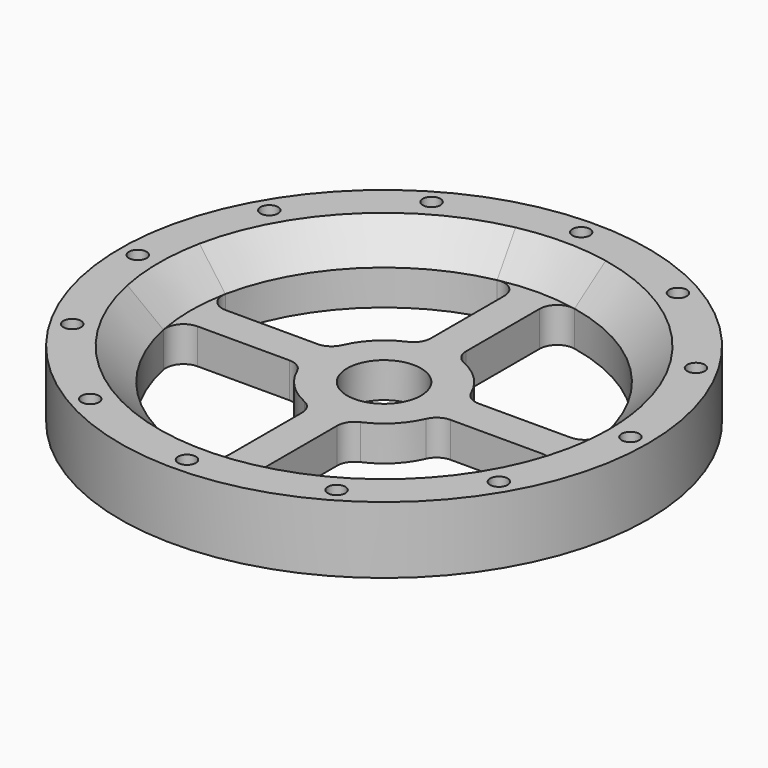
from build123d import *

# Parameters (mm, degrees)
F0_R     = 75
F0_R_2   = 2.5
F0_R_3   = 10.5
F1_DEPTH = 10
F2_R     = 5
F3_R     = 75
F3_R_2   = 2.5
F4_DEPTH = 9
F5_SIZE  = 8.99999


# Not quite as in the source:
# - a fillet or chamfer is up to 0.001 mm smaller than in the source, because OpenCascade refuses the exact size


with BuildPart() as f1:
    # F0 (on Top) → F1 (new body)
    with BuildSketch(Plane.XY):
        Circle(F0_R)
        with Locations((-35, -60.6217782649)):
            Circle(F0_R_2, mode=Mode.SUBTRACT)
        with Locations((-60.6217782649, -35)):
            Circle(F0_R_2, mode=Mode.SUBTRACT)
        with BuildLine():
            ThreePointArc((-5, -54.7722557505), (-38.8908729653, -38.8908729653), (-54.7722557505, -5))
            Line((-54.7722557505, -5), (-19.364916731, -5))
            ThreePointArc((-19.364916731, -5), (-14.1421356237, -14.1421356237), (-5, -19.364916731))
            Line((-5, -19.364916731), (-5, -54.7722557505))
        make_face(mode=Mode.SUBTRACT)
        with Locations((0, -70)):
            Circle(F0_R_2, mode=Mode.SUBTRACT)
        with Locations((35, -60.6217782649)):
            Circle(F0_R_2, mode=Mode.SUBTRACT)
        with BuildLine():
            Line((19.364916731, -5), (54.7722557505, -5))
            ThreePointArc((54.7722557505, -5), (38.8908729653, -38.8908729653), (5, -54.7722557505))
            Line((5, -54.7722557505), (5, -19.364916731))
            ThreePointArc((5, -19.364916731), (14.1421356237, -14.1421356237), (19.364916731, -5))
        make_face(mode=Mode.SUBTRACT)
        with Locations((60.6217782649, -35)):
            Circle(F0_R_2, mode=Mode.SUBTRACT)
        with Locations((-70, 0)):
            Circle(F0_R_2, mode=Mode.SUBTRACT)
        with Locations((-60.6217782649, 35)):
            Circle(F0_R_2, mode=Mode.SUBTRACT)
        with BuildLine():
            Line((-5, 54.7722557505), (-5, 19.364916731))
            ThreePointArc((-5, 19.364916731), (-14.1421356237, 14.1421356237), (-19.364916731, 5))
            Line((-19.364916731, 5), (-54.7722557505, 5))
            ThreePointArc((-54.7722557505, 5), (-38.8908729653, 38.8908729653), (-5, 54.7722557505))
        make_face(mode=Mode.SUBTRACT)
        with Locations((-35, 60.6217782649)):
            Circle(F0_R_2, mode=Mode.SUBTRACT)
        Circle(F0_R_3, mode=Mode.SUBTRACT)
        with BuildLine():
            ThreePointArc((5, 54.7722557505), (38.8908729653, 38.8908729653), (54.7722557505, 5))
            Line((54.7722557505, 5), (19.364916731, 5))
            ThreePointArc((19.364916731, 5), (14.1421356237, 14.1421356237), (5, 19.364916731))
            Line((5, 19.364916731), (5, 54.7722557505))
        make_face(mode=Mode.SUBTRACT)
        with Locations((70, 0)):
            Circle(F0_R_2, mode=Mode.SUBTRACT)
        with Locations((60.6217782649, 35)):
            Circle(F0_R_2, mode=Mode.SUBTRACT)
        with Locations((0, 70)):
            Circle(F0_R_2, mode=Mode.SUBTRACT)
        with Locations((35, 60.6217782649)):
            Circle(F0_R_2, mode=Mode.SUBTRACT)
    extrude(amount=F1_DEPTH)

    # F2
    f2_edges = [f1.edges().sort_by_distance(p)[0] for p in [
        (5, -54.772256, 5),
        (5, -19.364917, 5),
        (19.364917, -5, 5),
        (19.364917, 5, 5),
        (5, 19.364917, 5),
        (-5, 19.364917, 5),
        (-19.364917, 5, 5),
        (-5, -19.364917, 5),
        (-19.364917, -5, 5),
        (54.772256, 5, 5),
        (54.772256, -5, 5),
        (5, 54.772256, 5),
        (-54.772256, -5, 5),
        (-5, 54.772256, 5),
        (-5, -54.772256, 5),
        (-54.772256, 5, 5),
    ]]
    fillet(f2_edges, radius=F2_R)

    # F3 (on face) → F4 (join)
    with BuildSketch(Plane.XY.offset(10)):
        Circle(F3_R)
        with Locations((-35, -60.6217782649)):
            Circle(F3_R_2, mode=Mode.SUBTRACT)
        with Locations((-60.6217782649, -35)):
            Circle(F3_R_2, mode=Mode.SUBTRACT)
        with Locations((0, -70)):
            Circle(F3_R_2, mode=Mode.SUBTRACT)
        with Locations((35, -60.6217782649)):
            Circle(F3_R_2, mode=Mode.SUBTRACT)
        with Locations((60.6217782649, -35)):
            Circle(F3_R_2, mode=Mode.SUBTRACT)
        with Locations((-70, 0)):
            Circle(F3_R_2, mode=Mode.SUBTRACT)
        with Locations((-60.6217782649, 35)):
            Circle(F3_R_2, mode=Mode.SUBTRACT)
        with Locations((-35, 60.6217782649)):
            Circle(F3_R_2, mode=Mode.SUBTRACT)
        with BuildLine():
            ThreePointArc((53.8887743412, 11), (54.7214884153, 5.5279929103), (55, 0))
            ThreePointArc((55, 0), (54.7214884153, -5.5279929103), (53.8887743412, -11))
            ThreePointArc((53.8887743412, -11), (38.8908729653, -38.8908729653), (11, -53.8887743412))
            ThreePointArc((11, -53.8887743412), (0, -55), (-11, -53.8887743412))
            ThreePointArc((-11, -53.8887743412), (-38.8908729653, -38.8908729653), (-53.8887743412, -11))
            ThreePointArc((-53.8887743412, -11), (-55, 0), (-53.8887743412, 11))
            ThreePointArc((-53.8887743412, 11), (-38.8908729653, 38.8908729653), (-11, 53.8887743412))
            ThreePointArc((-11, 53.8887743412), (0, 55), (11, 53.8887743412))
            ThreePointArc((11, 53.8887743412), (38.8908729653, 38.8908729653), (53.8887743412, 11))
        make_face(mode=Mode.SUBTRACT)
        with Locations((70, 0)):
            Circle(F3_R_2, mode=Mode.SUBTRACT)
        with Locations((60.6217782649, 35)):
            Circle(F3_R_2, mode=Mode.SUBTRACT)
        with Locations((0, 70)):
            Circle(F3_R_2, mode=Mode.SUBTRACT)
        with Locations((35, 60.6217782649)):
            Circle(F3_R_2, mode=Mode.SUBTRACT)
    extrude(amount=F4_DEPTH)

    # F5 (size 9 in the source; OpenCascade refuses exactly that, so slightly less here)
    f5_edges = [f1.edges().sort_by_distance(p)[0] for p in [
        (53.888774, 11, 19),
    ]]
    chamfer(f5_edges, length=F5_SIZE)


solid = f1.part
